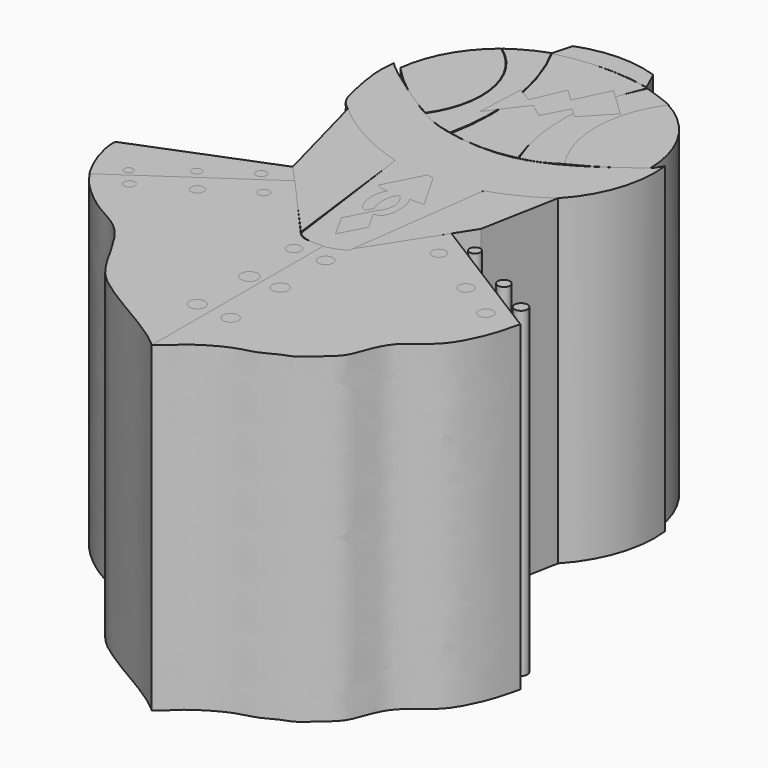
from build123d import *

# Parameters (mm, degrees)
F13_DEPTH = 50.8
F3_R      = 0.8258639316
F3_R_2    = 0.764978056
F3_R_3    = 0.6797787927
F3_R_4    = 0.8640740481
F3_R_5    = 0.9923388608
F3_R_6    = 0.8490565484
F3_R_7    = 1.1012910221
F3_R_8    = 1.1556611148
F3_R_9    = 1.2502681644
F3_R_10   = 1.3249013173
F3_R_11   = 1.1898830125
F3_R_12   = 1.2566568943
F3_R_13   = 0.8479964072
F3_R_14   = 1.0809877486
F3_R_15   = 1.1534001033
F3_R_16   = 0.9668649048
F3_R_17   = 1.0273458698
F3_R_18   = 1.137706782


# Not quite as in the source:
# - a feature of the source that left no trace in its solid (it failed there, or was rolled back) is left out


with BuildPart() as f13:
    # F9 (on Top) → F13 (new body)
    with BuildSketch(Plane.XY):
        with BuildLine():
            add(Edge.make_bspline(
                [(-21.125846708, 27.3723586698), (-20.8347521232, 27.1254879671), (-20.5297161329, 26.8714296714), (-20.2117994559, 26.6140409524)],
                knots=[0, 0, 0, 0, 0.031945991, 0.031945991, 0.031945991, 0.031945991], degree=3))
            ThreePointArc((-21.125846708, 27.3723586698), (-21.3344056847, 24.3224414992), (-20.8773446183, 21.2997627574))
            add(Edge.make_bspline(
                [(-20.8773446183, 21.2997627574), (-20.6619361674, 20.9767399348), (-20.4394229312, 20.6837653222), (-20.2117994559, 20.4157030891)],
                knots=[0, 0, 0, 0, 0.0250038431, 0.0250038431, 0.0250038431, 0.0250038431], degree=3))
            Line((-20.2117994559, 20.4157030891), (-20.2117994559, 26.6140409524))
        make_face()
        with BuildLine():
            add(Edge.make_bspline(
                [(-20.2117994559, 26.6140409524), (-19.904375261, 26.3651470584), (-19.5849065742, 26.1131389472), (-19.2543525186, 25.8615043496)],
                knots=[0.031945991, 0.031945991, 0.031945991, 0.031945991, 0.0628376406, 0.0628376406, 0.0628376406, 0.0628376406], degree=3))
            Line((-20.2117994559, 26.6140409524), (-20.2117994559, 20.4157030891))
            add(Edge.make_bspline(
                [(-20.2117994559, 20.4157030891), (-19.900507453, 20.0491080825), (-19.5796579779, 19.7291056859), (-19.2543525186, 19.4425598906)],
                knots=[0.0250038431, 0.0250038431, 0.0250038431, 0.0250038431, 0.059198455, 0.059198455, 0.059198455, 0.059198455], degree=3))
            Line((-19.2543525186, 19.4425598906), (-19.2543525186, 25.8615043496))
        make_face()
        with BuildLine():
            add(Edge.make_bspline(
                [(-19.2543525186, 25.8615043496), (-18.8314593105, 25.5395764818), (-18.3904223718, 25.2182599541), (-17.9332500512, 24.9048578725)],
                knots=[0.0628376406, 0.0628376406, 0.0628376406, 0.0628376406, 0.1023587675, 0.1023587675, 0.1023587675, 0.1023587675], degree=3))
            Line((-19.2543525186, 25.8615043496), (-19.2543525186, 19.4425598906))
            add(Edge.make_bspline(
                [(-19.2543525186, 19.4425598906), (-18.817899269, 19.0581093996), (-18.3734248739, 18.7338835997), (-17.9332500512, 18.4381574226)],
                knots=[0.059198455, 0.059198455, 0.059198455, 0.059198455, 0.1050764107, 0.1050764107, 0.1050764107, 0.1050764107], degree=3))
            Line((-17.9332500512, 18.4381574226), (-17.9332500512, 24.9048578725))
        make_face()
        with BuildLine():
            add(Edge.make_bspline(
                [(-17.9332500512, 24.9048578725), (-17.3830906612, 24.5277110282), (-16.8095646212, 24.1620255855), (-16.2161719054, 23.8205287606)],
                knots=[0.1023587675, 0.1023587675, 0.1023587675, 0.1023587675, 0.1499183376, 0.1499183376, 0.1499183376, 0.1499183376], degree=3))
            Line((-17.9332500512, 24.9048578725), (-17.9332500512, 18.4381574226))
            add(Edge.make_bspline(
                [(-17.9332500512, 18.4381574226), (-17.6086585708, 18.2200845282), (-17.0105720145, 17.8441146508), (-16.4375567591, 17.4777070139), (-16.1744944867, 17.3109124212)],
                knots=[0.1050764107, 0.1050764107, 0.1050764107, 0.1050764107, 0.1389074997, 0.1678652471, 0.1678652471, 0.1678652471, 0.1678652471], degree=3))
            Line((-16.1744944867, 17.3109124212), (-16.2161719054, 23.8205287606))
        make_face()
        with BuildLine():
            add(Edge.make_bspline(
                [(-16.2161719054, 23.8205287606), (-16.0014371982, 23.6969491837), (-15.5601814874, 23.452478006), (-15.1088853591, 23.2235501025), (-14.8776807746, 23.1111352228)],
                knots=[0.1499183376, 0.1499183376, 0.1499183376, 0.1499183376, 0.1671290147, 0.1848609969, 0.1848609969, 0.1848609969, 0.1848609969], degree=3))
            Line((-16.2161719054, 23.8205287606), (-16.1744944867, 17.3109124212))
            add(Edge.make_bspline(
                [(-16.1744944867, 17.3109124212), (-15.7449865853, 17.0385830032), (-15.3186992984, 16.7720913944), (-14.8776807746, 16.5121166992)],
                knots=[0.1678652471, 0.1678652471, 0.1678652471, 0.1678652471, 0.215145236, 0.215145236, 0.215145236, 0.215145236], degree=3))
            Line((-14.8776807746, 16.5121166992), (-14.8776807746, 23.1111352228))
        make_face()
        with BuildLine():
            add(Edge.make_bspline(
                [(-14.8776807746, 23.1111352228), (-14.3070567596, 22.8336899024), (-13.7230922448, 22.5791279001), (-13.1317322997, 22.3437527448)],
                knots=[0.1848609969, 0.1848609969, 0.1848609969, 0.1848609969, 0.2286243804, 0.2286243804, 0.2286243804, 0.2286243804], degree=3))
            Line((-14.8776807746, 23.1111352228), (-14.8776807746, 16.5121166992))
            add(Edge.make_bspline(
                [(-14.8776807746, 16.5121166992), (-14.4636429412, 16.2680467708), (-13.8984861896, 15.9526259429), (-13.2845672983, 15.648250525), (-13.1317322997, 15.574692191)],
                knots=[0.215145236, 0.215145236, 0.215145236, 0.215145236, 0.2595327234, 0.2738913967, 0.2738913967, 0.2738913967, 0.2738913967], degree=3))
            Line((-13.1317322997, 15.574692191), (-13.1317322997, 22.3437527448))
        make_face()
        with BuildLine():
            add(Edge.make_bspline(
                [(-13.1317322997, 22.3437527448), (-12.5834968737, 22.1255421615), (-12.0289053022, 21.9238220846), (-11.4726945758, 21.7356471914)],
                knots=[0.2286243804, 0.2286243804, 0.2286243804, 0.2286243804, 0.2691963491, 0.2691963491, 0.2691963491, 0.2691963491], degree=3))
            Line((-13.1317322997, 22.3437527448), (-13.1317322997, 15.574692191))
            add(Edge.make_bspline(
                [(-13.1317322997, 15.574692191), (-12.6094536829, 15.3233234257), (-12.0546922141, 15.0817263388), (-11.4726945758, 14.8569610447)],
                knots=[0.2738913967, 0.2738913967, 0.2738913967, 0.2738913967, 0.3229588757, 0.3229588757, 0.3229588757, 0.3229588757], degree=3))
            Line((-11.4726945758, 14.8569610447), (-11.4726945758, 21.7356471914))
        make_face()
        with BuildLine():
            add(Edge.make_bspline(
                [(-11.4726945758, 21.7356471914), (-10.8241176286, 21.5162233436), (-10.1733391103, 21.3152169328), (-9.5278695226, 21.1279581478)],
                knots=[0.2691963491, 0.2691963491, 0.2691963491, 0.2691963491, 0.3165058352, 0.3165058352, 0.3165058352, 0.3165058352], degree=3))
            Line((-11.4726945758, 21.7356471914), (-11.4726945758, 14.8569610447))
            add(Edge.make_bspline(
                [(-11.4726945758, 14.8569610447), (-10.853171685, 14.6177036395), (-10.2027872041, 14.3975185158), (-9.5278695226, 14.2049213694)],
                knots=[0.3229588757, 0.3229588757, 0.3229588757, 0.3229588757, 0.3751900608, 0.3751900608, 0.3751900608, 0.3751900608], degree=3))
            Line((-9.5278695226, 14.2049213694), (-9.5278695226, 21.1279581478))
        make_face()
        with BuildLine():
            add(Edge.make_bspline(
                [(-9.5278695226, 21.1279581478), (-9.1488679975, 21.0180050742), (-8.5926706461, 20.862851759), (-8.0437599408, 20.7159498258), (-7.8676519915, 20.6696810568)],
                knots=[0.3165058352, 0.3165058352, 0.3165058352, 0.3165058352, 0.3442846302, 0.3574699751, 0.3574699751, 0.3574699751, 0.3574699751], degree=3))
            Line((-9.5278695226, 21.1279581478), (-9.5278695226, 14.2049213694))
            add(Edge.make_bspline(
                [(-9.5278695226, 14.2049213694), (-9.2039090788, 14.1124747514), (-8.6556599801, 13.9692796344), (-8.0937090418, 13.8462753142), (-7.8676519915, 13.8003926225)],
                knots=[0.3751900608, 0.3751900608, 0.3751900608, 0.3751900608, 0.4002610263, 0.4168909002, 0.4168909002, 0.4168909002, 0.4168909002], degree=3))
            Line((-7.8676519915, 13.8003926225), (-7.8676519915, 20.6696810568))
        make_face()
        with BuildLine():
            add(Edge.make_bspline(
                [(-7.8676519915, 20.6696810568), (-7.4364796265, 20.5563993186), (-7.0087411364, 20.449203879), (-6.5817643521, 20.3504497102)],
                knots=[0.3574699751, 0.3574699751, 0.3574699751, 0.3574699751, 0.3897521995, 0.3897521995, 0.3897521995, 0.3897521995], degree=3))
            Line((-7.8676519915, 20.6696810568), (-7.8676519915, 13.8003926225))
            add(Edge.make_bspline(
                [(-7.8676519915, 13.8003926225), (-7.2935890267, 13.6838753365), (-6.7069076556, 13.5878021605), (-6.1112494197, 13.511504583)],
                knots=[0.4168909002, 0.4168909002, 0.4168909002, 0.4168909002, 0.459121809, 0.459121809, 0.459121809, 0.459121809], degree=3))
            Line((-6.1112494197, 13.511504583), (-6.5817643521, 20.3504497102))
        make_face()
        with BuildLine():
            add(Edge.make_bspline(
                [(-6.5817643521, 20.3504497102), (-6.0578024629, 20.22926415), (-5.5349876125, 20.1207901455), (-5.0083818106, 20.0293795287)],
                knots=[0.3897521995, 0.3897521995, 0.3897521995, 0.3897521995, 0.4293671292, 0.4293671292, 0.4293671292, 0.4293671292], degree=3))
            Line((-6.5817643521, 20.3504497102), (-6.1112494197, 13.511504583))
            add(Edge.make_bspline(
                [(-6.1112494197, 13.511504583), (-5.62787322, 13.4495891576), (-5.1385854764, 13.4006965769), (-4.6453322191, 13.3644695901)],
                knots=[0.459121809, 0.459121809, 0.459121809, 0.459121809, 0.493392159, 0.493392159, 0.493392159, 0.493392159], degree=3))
            Line((-4.6453322191, 13.3644695901), (-5.0083818106, 20.0293795287))
        make_face()
        with BuildLine():
            add(Edge.make_bspline(
                [(-5.0083818106, 20.0293795287), (-4.4190508025, 19.927080787), (-3.8249719601, 19.846152441), (-3.2192242461, 19.7926939744)],
                knots=[0.4293671292, 0.4293671292, 0.4293671292, 0.4293671292, 0.4737006826, 0.4737006826, 0.4737006826, 0.4737006826], degree=3))
            Line((-5.0083818106, 20.0293795287), (-4.6453322191, 13.3644695901))
            add(Edge.make_bspline(
                [(-4.6453322191, 13.3644695901), (-4.0948822571, 13.3240417912), (-3.5394937933, 13.2993872473), (-2.9818713665, 13.2900094613)],
                knots=[0.493392159, 0.493392159, 0.493392159, 0.493392159, 0.5316364333, 0.5316364333, 0.5316364333, 0.5316364333], degree=3))
            Line((-2.9818713665, 13.2900094613), (-3.2192242461, 19.7926939744))
        make_face()
        with BuildLine():
            add(Edge.make_bspline(
                [(-3.2192242461, 19.7926939744), (-2.6894172346, 19.7459374292), (-2.1506837335, 19.7201948771), (-1.5983930182, 19.719547358)],
                knots=[0.4737006826, 0.4737006826, 0.4737006826, 0.4737006826, 0.5124762766, 0.5124762766, 0.5124762766, 0.5124762766], degree=3))
            Line((-3.2192242461, 19.7926939744), (-2.9818713665, 13.2900094613))
            add(Edge.make_bspline(
                [(-2.9818713665, 13.2900094613), (-2.598295297, 13.2835586909), (-2.0336888013, 13.2847004629), (-1.4687014205, 13.3010698813), (-1.288695996, 13.3077850564)],
                knots=[0.5316364333, 0.5316364333, 0.5316364333, 0.5316364333, 0.5579438193, 0.5702532866, 0.5702532866, 0.5702532866, 0.5702532866], degree=3))
            Line((-1.288695996, 13.3077850564), (-1.5983930182, 19.719547358))
        make_face()
        with BuildLine():
            add(Edge.make_bspline(
                [(-1.5983930182, 19.719547358), (-1.0760239175, 19.7189349198), (-0.541526796, 19.7407720111), (0, 19.7822179046)],
                knots=[0.5124762766, 0.5124762766, 0.5124762766, 0.5124762766, 0.549151114, 0.549151114, 0.549151114, 0.549151114], degree=3))
            Line((-1.5983930182, 19.719547358), (-1.288695996, 13.3077850564))
            add(Edge.make_bspline(
                [(-1.288695996, 13.3077850564), (-0.7545655199, 13.3277110099), (-0.2212218042, 13.3608203078), (0.3079894723, 13.4058075855)],
                knots=[0.5702532866, 0.5702532866, 0.5702532866, 0.5702532866, 0.6067791948, 0.6067791948, 0.6067791948, 0.6067791948], degree=3))
            Line((0.3079894723, 13.4058075855), (0, 19.7822179046))
        make_face()
        with BuildLine():
            add(Edge.make_bspline(
                [(0, 19.7822179046), (0.5137068711, 19.8215345929), (1.0337396967, 19.878497104), (1.5557462092, 19.950680415)],
                knots=[0.549151114, 0.549151114, 0.549151114, 0.549151114, 0.5839418503, 0.5839418503, 0.5839418503, 0.5839418503], degree=3))
            Line((0, 19.7822179046), (0.3079894723, 13.4058075855))
            add(Edge.make_bspline(
                [(0.3079894723, 13.4058075855), (0.7270533852, 13.4414314383), (1.143526051, 13.4845033813), (1.5557462092, 13.5343752499)],
                knots=[0.6067791948, 0.6067791948, 0.6067791948, 0.6067791948, 0.6357027849, 0.6357027849, 0.6357027849, 0.6357027849], degree=3))
            Line((1.5557462092, 13.5343752499), (1.5557462092, 19.950680415))
        make_face()
        with BuildLine():
            add(Edge.make_bspline(
                [(1.5557462092, 19.950680415), (2.0910865169, 20.0247075295), (2.6285026284, 20.1147429555), (3.16330017, 20.2181710532)],
                knots=[0.5839418503, 0.5839418503, 0.5839418503, 0.5839418503, 0.6196212585, 0.6196212585, 0.6196212585, 0.6196212585], degree=3))
            Line((1.5557462092, 19.950680415), (1.5557462092, 13.5343752499))
            add(Edge.make_bspline(
                [(1.5557462092, 13.5343752499), (2.1002950478, 13.6002567153), (2.6374229225, 13.6780045916), (3.16330017, 13.7661246805)],
                knots=[0.6357027849, 0.6357027849, 0.6357027849, 0.6357027849, 0.673911269, 0.673911269, 0.673911269, 0.673911269], degree=3))
            Line((3.16330017, 13.7661246805), (3.16330017, 20.2181710532))
        make_face()
        with BuildLine():
            add(Edge.make_bspline(
                [(3.16330017, 20.2181710532), (3.8146725961, 20.3441443529), (4.4621604418, 20.4899853328), (5.0972817207, 20.6509679486)],
                knots=[0.6196212585, 0.6196212585, 0.6196212585, 0.6196212585, 0.6630780453, 0.6630780453, 0.6630780453, 0.6630780453], degree=3))
            Line((3.16330017, 20.2181710532), (3.16330017, 13.7661246805))
            add(Edge.make_bspline(
                [(3.16330017, 13.7661246805), (3.7296270842, 13.8610228308), (4.2829060457, 13.9679501896), (4.818353959, 14.0850405636)],
                knots=[0.673911269, 0.673911269, 0.673911269, 0.673911269, 0.7150586908, 0.7150586908, 0.7150586908, 0.7150586908], degree=3))
            Line((4.818353959, 14.0850405636), (5.0972817207, 20.6509679486))
        make_face()
        with BuildLine():
            add(Edge.make_bspline(
                [(5.0972817207, 20.6509679486), (5.58535494, 20.7746786573), (6.0661250841, 20.9073312582), (6.5357428463, 21.0467809712)],
                knots=[0.6630780453, 0.6630780453, 0.6630780453, 0.6630780453, 0.6964733896, 0.6964733896, 0.6964733896, 0.6964733896], degree=3))
            Line((5.0972817207, 20.6509679486), (4.818353959, 14.0850405636))
            add(Edge.make_bspline(
                [(4.818353959, 14.0850405636), (5.3750991504, 14.2067881717), (5.9125666354, 14.3395233348), (6.4412617638, 14.4826543305)],
                knots=[0.7150586908, 0.7150586908, 0.7150586908, 0.7150586908, 0.7578427388, 0.7578427388, 0.7578427388, 0.7578427388], degree=3))
            Line((6.4412617638, 14.4826543305), (6.5357428463, 21.0467809712))
        make_face()
        with BuildLine():
            add(Edge.make_bspline(
                [(6.5357428463, 21.0467809712), (7.1170989648, 21.2194106083), (7.6813642554, 21.4024566995), (8.2282215408, 21.5939352841)],
                knots=[0.6964733896, 0.6964733896, 0.6964733896, 0.6964733896, 0.7378146449, 0.7378146449, 0.7378146449, 0.7378146449], degree=3))
            Line((6.5357428463, 21.0467809712), (6.4412617638, 14.4826543305))
            add(Edge.make_bspline(
                [(6.4412617638, 14.4826543305), (6.9056378419, 14.6083725504), (7.3632461539, 14.7421110284), (7.8212054558, 14.8834687947)],
                knots=[0.7578427388, 0.7578427388, 0.7578427388, 0.7578427388, 0.7954218413, 0.7954218413, 0.7954218413, 0.7954218413], degree=3))
            Line((7.8212054558, 14.8834687947), (8.2282215408, 21.5939352841))
        make_face()
        with BuildLine():
            add(Edge.make_bspline(
                [(8.2282215408, 21.5939352841), (8.6633628548, 21.746297235), (9.0874821375, 21.9039982932), (9.500419591, 22.0660389143)],
                knots=[0.7378146449, 0.7378146449, 0.7378146449, 0.7378146449, 0.7707104087, 0.7707104087, 0.7707104087, 0.7707104087], degree=3))
            Line((8.2282215408, 21.5939352841), (7.8212054558, 14.8834687947))
            add(Edge.make_bspline(
                [(7.8212054558, 14.8834687947), (8.5874074933, 15.1199714884), (9.6396761943, 15.4736113373), (10.7565133697, 15.8638421146), (11.0588213429, 15.9738352262)],
                knots=[0.7954218413, 0.7954218413, 0.7954218413, 0.7954218413, 0.8582946442, 0.881658047, 0.881658047, 0.881658047, 0.881658047], degree=3))
            Line((11.0588213429, 15.9738352262), (11.0588213429, 22.7200354778))
            add(Edge.make_bspline(
                [(9.500419591, 22.0660389143), (10.0390285895, 22.2773942561), (10.5586140402, 22.4961324584), (11.0588213429, 22.7200354778)],
                knots=[0.7707104087, 0.7707104087, 0.7707104087, 0.7707104087, 0.8136175228, 0.8136175228, 0.8136175228, 0.8136175228], degree=3))
        make_face()
        with BuildLine():
            Line((11.0588213429, 22.7200354778), (11.0588213429, 15.9738352262))
            add(Edge.make_bspline(
                [(11.0588213429, 15.9738352262), (11.5241048545, 16.1431261011), (11.9887504135, 16.3225330625), (12.434497183, 16.5178338427)],
                knots=[0.881658047, 0.881658047, 0.881658047, 0.881658047, 0.9176167616, 0.9176167616, 0.9176167616, 0.9176167616], degree=3))
            Line((12.434497183, 16.5178338427), (12.6337970085, 23.4722221968))
            add(Edge.make_bspline(
                [(11.0588213429, 22.7200354778), (11.6072647333, 22.9655299566), (12.1324124203, 23.2172333904), (12.6337970085, 23.4722221968)],
                knots=[0.8136175228, 0.8136175228, 0.8136175228, 0.8136175228, 0.8606622641, 0.8606622641, 0.8606622641, 0.8606622641], degree=3))
        make_face()
        with BuildLine():
            Line((12.6337970085, 23.4722221968), (12.434497183, 16.5178338427))
            add(Edge.make_bspline(
                [(12.434497183, 16.5178338427), (12.8998213773, 16.7217123326), (13.3445502373, 16.9429114299), (13.7479096275, 17.1880040753)],
                knots=[0.9176167616, 0.9176167616, 0.9176167616, 0.9176167616, 0.9551548011, 0.9551548011, 0.9551548011, 0.9551548011], degree=3))
            Line((13.7479096275, 17.1880040753), (14.17928578, 24.3000945385))
            add(Edge.make_bspline(
                [(12.6337970085, 23.4722221968), (13.1713354673, 23.7455977515), (13.6815602475, 24.0227495651), (14.17928578, 24.3000945385)],
                knots=[0.8606622641, 0.8606622641, 0.8606622641, 0.8606622641, 0.9110993104, 0.9110993104, 0.9110993104, 0.9110993104], degree=3))
        make_face()
        with BuildLine():
            Line((14.17928578, 24.3000945385), (13.7479096275, 17.1880040753))
            add(Edge.make_bspline(
                [(13.7479096275, 17.1880040753), (14.2297870054, 17.4808064848), (14.6526213462, 17.8077100721), (14.980992038, 18.179921926)],
                knots=[0.9551548011, 0.9551548011, 0.9551548011, 0.9551548011, 1, 1, 1, 1], degree=3))
            Line((14.980992038, 18.179921926), (15.3937334453, 24.9847816969))
            add(Edge.make_bspline(
                [(14.17928578, 24.3000945385), (14.5898345398, 24.5288624587), (14.9918790985, 24.7577618003), (15.3937334453, 24.9847816969)],
                knots=[0.9110993104, 0.9110993104, 0.9110993104, 0.9110993104, 0.9527022933, 0.9527022933, 0.9527022933, 0.9527022933], degree=3))
        make_face()
        with BuildLine():
            Line((15.3937334453, 24.9847816969), (14.980992038, 18.179921926))
            ThreePointArc((14.980992038, 18.179921926), (16.5063806562, 21.8154594304), (16.7757962894, 25.7488242238))
            add(Edge.make_bspline(
                [(15.3937334453, 24.9847816969), (15.8505946536, 25.2428766637), (16.3072100126, 25.4985424439), (16.7757962894, 25.7488242238)],
                knots=[0.9527022933, 0.9527022933, 0.9527022933, 0.9527022933, 1, 1, 1, 1], degree=3))
        make_face()
    extrude(amount=F13_DEPTH)


with BuildPart() as f13b:
    # F8 (on Top) → F13, piece 2 (new body)
    with BuildSketch(Plane.XY):
        with BuildLine():
            ThreePointArc((-12.3988108372, 23.6741252104), (-10.1171786146, 33.994784483), (-15.8344633881, 42.8849199285))
            ThreePointArc((-15.8344633881, 42.8849199285), (-20.2435563178, 37.6436153683), (-22.3273675175, 31.1191150167))
            ThreePointArc((-22.3273675175, 31.1191150167), (-17.6977421328, 26.9503306057), (-12.3988108372, 23.6741252104))
        make_face()
    extrude(amount=F13_DEPTH)


with BuildPart() as f13c:
    # F8 (on Top) → F13, piece 3 (new body)
    with BuildSketch(Plane.XY):
        with BuildLine():
            ThreePointArc((9.5350146294, 44.1038645804), (6.257298337, 33.888541162), (9.5350146294, 23.6732177436))
            ThreePointArc((9.5350146294, 23.6732177436), (14.177280096, 26.3004344114), (18.5024803593, 29.4222189595))
            ThreePointArc((18.5024803593, 29.4222189595), (16.0429971981, 37.999441988), (9.5350146294, 44.1038645804))
        make_face()
    extrude(amount=F13_DEPTH)


with BuildPart() as f13d:
    # F8 (on Top) → F13, piece 4 (new body)
    with BuildSketch(Plane.XY):
        with BuildLine():
            ThreePointArc((-10.1647363602, 45.9095185055), (-6.1837471128, 33.9589399996), (-6.5014758147, 21.3667340577))
            ThreePointArc((-6.5014758147, 21.3667340577), (-1.2340764428, 20.7648960213), (4.0342169814, 21.3588569313))
            ThreePointArc((4.0342169814, 21.3588569313), (2.0273038958, 33.7407666562), (4.8860239137, 45.9541653817))
            ThreePointArc((4.8860239137, 45.9541653817), (-2.6417550196, 46.7404922067), (-10.1647363602, 45.9095185055))
        make_face()
    extrude(amount=F13_DEPTH)


with BuildPart() as f13e:
    # F7 (on Top) → F13, piece 5 (new body)
    with BuildSketch(Plane.XY):
        with BuildLine():
            ThreePointArc((-12.3944459483, 23.4615169466), (-9.6503858131, 22.2226681718), (-6.7442338914, 21.4359704405))
            ThreePointArc((-6.7442338914, 21.4359704405), (-6.2858776286, 33.9589836539), (-10.2293472737, 45.8537302911))
            ThreePointArc((-10.2293472737, 45.8537302911), (-13.0947819539, 44.6092461951), (-15.7425962389, 42.951375246))
            ThreePointArc((-15.7425962389, 42.951375246), (-10.0041611915, 33.9046598841), (-12.3944459483, 23.4615169466))
        make_face()
    extrude(amount=F13_DEPTH)


with BuildPart() as f13f:
    # F7 (on Top) → F13, piece 6 (new body)
    with BuildSketch(Plane.XY):
        with BuildLine():
            ThreePointArc((9.7108701983, 44.0882421106), (7.3439136897, 45.0182369237), (4.9339610864, 45.8303341562))
            ThreePointArc((4.9339610864, 45.8303341562), (1.9006592019, 33.6722260465), (4.1810232215, 21.3506817818))
            ThreePointArc((4.1810232215, 21.3506817818), (6.9727148218, 22.2661082897), (9.5312194899, 23.7102694809))
            ThreePointArc((9.5312194899, 23.7102694809), (6.4216220228, 33.9274616721), (9.7108701983, 44.0882421106))
        make_face()
    extrude(amount=F13_DEPTH)


with BuildPart() as f13g:
    # F11 (on Top) → F13, piece 7 (new body)
    with BuildSketch(Plane.XY):
        with BuildLine():
            ThreePointArc((-7.3326835409, 11.3885579631), (-14.377405186, 14.2696952056), (-20.5801893026, 18.6804234982))
            Line((-20.5801893026, 18.6804234982), (-16.1750596017, 2.1767148282))
            Line((-16.1750596017, 2.1767148282), (-4.507355392, -10.7746338472))
            Line((-4.507355392, -10.7746338472), (-7.3326835409, 11.3885579631))
        make_face()
    extrude(amount=F13_DEPTH)


with BuildPart() as f13h:
    # F11 (on Top) → F13, piece 8 (new body)
    with BuildSketch(Plane.XY):
        with BuildLine():
            Line((6.2384190969, 11.8528539315), (3.1280014664, -10.5955125764))
            Line((3.1280014664, -10.5955125764), (12.3193198815, 3.711481113))
            Line((12.3193198815, 3.711481113), (14.6430647001, 16.0904526711))
            ThreePointArc((14.6430647001, 16.0904526711), (10.586652774, 13.6822608237), (6.2384190969, 11.8528539315))
        make_face()
    extrude(amount=F13_DEPTH)


with BuildPart() as f13i:
    # F6 (on Top) → F13, piece 9 (new body)
    with BuildSketch(Plane.XY):
        with BuildLine():
            add(Edge.make_bspline(
                [(0, -12.0247779414), (0.5012354918, -11.9426944258), (1.7908691638, -11.7338985108), (2.6501969117, -11.1655605144), (3.1240915414, -10.5731924996)],
                knots=[0, 0, 0, 0, 0.492792412, 1, 1, 1, 1], degree=3))
            Line((0, -12.0247779414), (0, -45.9450371563))
            add(Edge.make_bspline(
                [(32.0461690426, -13.1501732394), (31.7097565093, -14.5282364317), (31.0642043992, -17.3739063034), (28.646181352, -22.4797561646), (26.1181511575, -24.640107946), (22.9830511449, -26.8576842658), (21.4926242295, -30.1016614383), (20.5465442347, -33.3459081143), (17.8988820449, -35.3011340828), (15.9446171515, -37.3481670644), (13.8112930921, -37.899895011), (11.542638481, -39.3912219109), (8.5051505152, -39.9352404708), (5.444791947, -41.5575600393), (2.4923123567, -43.5404964495), (1.700661544, -44.6719397288), (0, -45.9450371563)],
                knots=[0, 0, 0, 0, 0.0814586936, 0.1723459536, 0.2433655723, 0.3178750274, 0.3907644345, 0.4610811587, 0.5307268637, 0.5952181363, 0.6517409884, 0.7147459782, 0.782686328, 0.8556077005, 0.924329985, 1, 1, 1, 1], degree=3))
            Line((32.0461690426, -13.1501732394), (10.2511029691, 0.4863103968))
            Line((10.2511029691, 0.4863103968), (3.1240915414, -10.5731924996))
        make_face()
    extrude(amount=F13_DEPTH)


with BuildPart() as f13j:
    # F12 (on Top) → F13, piece 10 (new body)
    with BuildSketch(Plane.XY):
        with BuildLine():
            add(Edge.make_bspline(
                [(-23.7491764128, 31.6212512553), (-23.5014987322, 31.3483771554), (-22.5627618935, 30.3140691193), (-12.0611662049, 22.8982617788), (-7.0474683792, 21.2085651947), (5.2835711864, 19.5360643586), (14.377356866, 26.3330175771), (18.7600348145, 29.6710412949)],
                knots=[0, 0, 0, 0, 0.0861918774, 0.3258221147, 0.4937836066, 0.720934999, 1, 1, 1, 1], degree=3))
            add(Edge.make_bspline(
                [(-23.7491764128, 31.6212512553), (-23.8477742303, 30.5311013084), (-24.067282785, 28.1040979001), (-23.0487521074, 22.9537554354), (-22.3178278064, 19.9419018956), (-21.1057583084, 18.9667539886), (-20.5545537174, 18.523292616)],
                knots=[0, 0, 0, 0, 0.2545070369, 0.566609619, 0.8029100079, 1, 1, 1, 1], degree=3))
            ThreePointArc((-20.5545537174, 18.523292616), (-14.3465072066, 14.2264422516), (-7.3501081206, 11.3886324689))
            Line((-7.3501081206, 11.3886324689), (-4.3249502778, -10.8443647623))
            add(Edge.make_bspline(
                [(-4.3249502778, -10.8443647623), (-3.9669240627, -11.6108496135), (-1.9831716654, -12.1008701365), (-0.1800869966, -12.2315672406), (2.1804859454, -11.5264114101), (1.6686771996, -11.6793001071), (3.211584175, -10.8443647623)],
                knots=[0, 0, 0, 0, 0.2802837955, 0.5352435302, 0.7663564293, 1, 1, 1, 1], degree=3))
            Line((3.211584175, -10.8443647623), (6.2316702679, 11.8567077443))
            ThreePointArc((6.2316702679, 11.8567077443), (10.5869107262, 13.6279285619), (14.6170314401, 16.0493887961))
            ThreePointArc((14.6170314401, 16.0493887961), (18.7520084952, 22.9933533972), (19.5831675082, 31.0323741287))
            Line((19.5831675082, 31.0323741287), (18.7600348145, 29.6710412949))
        make_face()
    extrude(amount=F13_DEPTH)


with BuildPart() as f13k:
    # F1 (on Top) → F13, piece 11 (new body)
    with BuildSketch(Plane.XY):
        Polygon((6.5561048687, 38.4634584188), (2.0181094296, 42.7997633815), (-0.5179300206, 37.5159755349), (-2.4259227794, 39.3815711141), (-4.6731135808, 34.33545), (-7.0475041866, 35.8129740924), (-7.3556074226, 28.1221466535), (-3.2739192247, 33.5303917527), (-1.0267283069, 31.8344011903), (1.0653183376, 35.8129740924), (2.6115651192, 34.33545), align=None)
    extrude(amount=F13_DEPTH)


with BuildPart() as f13l:
    # F2 (on Top) → F13, piece 12 (new body)
    with BuildSketch(Plane.XY):
        with BuildLine():
            Line((4.6263667755, 46.0232459009), (3.2002124935, 49.1607859731))
            ThreePointArc((3.2002124935, 49.1607859731), (-3.0867123745, 50.140822554), (-9.3360953033, 48.9445328712))
            Line((-9.3360953033, 48.9445328712), (-10.2056413889, 45.7380153239))
            ThreePointArc((-10.2056413889, 45.7380153239), (-2.8065800825, 46.7616560321), (4.6263667755, 46.0232459009))
        make_face()
    extrude(amount=F13_DEPTH)


with BuildPart() as f13m:
    # F4 (on Top) → F13, piece 13 (new body)
    with BuildSketch(Plane.XY):
        with BuildLine():
            Line((-34.5214679837, -15.0747038424), (-13.6476866901, -0.6190927234))
            Line((-13.6476866901, -0.6190927234), (-16.1745920777, 2.1744580008))
            Line((-16.1745920777, 2.1744580008), (-37.4110601842, -6.274796091))
            add(Edge.make_bspline(
                [(-34.5214679837, -15.0747038424), (-34.8318337722, -14.6441931803), (-35.4131860958, -13.573033533), (-36.7515156736, -10.8689685545), (-37.5907054956, -7.3068456647), (-37.4076562249, -6.5654079293), (-37.4110601842, -6.274796091)],
                knots=[0, 0, 0, 0, 0.2169891206, 0.5159779156, 0.8345383602, 1, 1, 1, 1], degree=3))
        make_face()
    extrude(amount=F13_DEPTH)


with BuildPart() as f13n:
    # F5 (on Top) → F13, piece 14 (new body)
    with BuildSketch(Plane.XY):
        with BuildLine():
            Line((0, -45.8658896387), (0, -11.98398415))
            add(Edge.make_bspline(
                [(0, -11.98398415), (-0.757853317, -12.0691313531), (-2.2823968877, -11.9373347854), (-3.522585379, -11.98398415), (-4.4776955619, -10.8777750283)],
                knots=[0, 0, 0, 0, 0.4771596755, 1, 1, 1, 1], degree=3))
            Line((-4.4776955619, -10.8777750283), (-13.6284315959, -0.5788833369))
            Line((-13.6284315959, -0.5788833369), (-34.5914363861, -14.926860109))
            add(Edge.make_bspline(
                [(0, -45.8658896387), (-1.0862513072, -44.8902953717), (-3.5963360104, -43.0816351518), (-7.4779805105, -40.839725523), (-13.8657304028, -37.0070267492), (-16.9276314083, -34.3148966756), (-19.6071658184, -29.5579111833), (-22.7281685987, -23.9817210793), (-27.1986720795, -21.8033968956), (-29.9162115543, -19.9481899875), (-32.9156425637, -17.3024699024), (-34.0417535859, -15.6896636097), (-34.5914363861, -14.926860109)],
                knots=[0, 0, 0, 0, 0.0976146874, 0.1981798717, 0.3239604974, 0.4180537563, 0.5254412879, 0.6429781982, 0.744207795, 0.8290483984, 0.9208484418, 1, 1, 1, 1], degree=3))
        make_face()
    extrude(amount=F13_DEPTH)


with BuildPart() as f13o:
    # F3 (on Top) → F13, piece 15 (new body)
    with BuildSketch(Plane.XY):
        with Locations((-18.0757213384, -1.6571147135)):
            Circle(F3_R)
    extrude(amount=F13_DEPTH)


with BuildPart() as f13p:
    # F3 (on Top) → F13, piece 16 (new body)
    with BuildSketch(Plane.XY):
        with Locations((-24.6791169047, -6.1492202803)):
            Circle(F3_R_2)
    extrude(amount=F13_DEPTH)


with BuildPart() as f13q:
    # F3 (on Top) → F13, piece 17 (new body)
    with BuildSketch(Plane.XY):
        with Locations((-31.4172767103, -11.1803784966)):
            Circle(F3_R_3)
    extrude(amount=F13_DEPTH)


with BuildPart() as f13r:
    # F3 (on Top) → F13, piece 18 (new body)
    with BuildSketch(Plane.XY):
        with Locations((-14.6617209539, -5.4330052808)):
            Circle(F3_R_4)
    extrude(amount=F13_DEPTH)


with BuildPart() as f13s:
    # F3 (on Top) → F13, piece 19 (new body)
    with BuildSketch(Plane.XY):
        with Locations((-21.5795636177, -9.8801897839)):
            Circle(F3_R_5)
    extrude(amount=F13_DEPTH)


with BuildPart() as f13t:
    # F3 (on Top) → F13, piece 20 (new body)
    with BuildSketch(Plane.XY):
        with Locations((-29.0500540286, -13.9810964465)):
            Circle(F3_R_6)
    extrude(amount=F13_DEPTH)


with BuildPart() as f13u:
    # F3 (on Top) → F13, piece 21 (new body)
    with BuildSketch(Plane.XY):
        with Locations((-2.3890119046, -14.7747769952)):
            Circle(F3_R_7)
    extrude(amount=F13_DEPTH)


with BuildPart() as f13v:
    # F3 (on Top) → F13, piece 22 (new body)
    with BuildSketch(Plane.XY):
        with Locations((2.6325094514, -14.8281967267)):
            Circle(F3_R_8)
    extrude(amount=F13_DEPTH)


with BuildPart() as f13w:
    # F3 (on Top) → F13, piece 23 (new body)
    with BuildSketch(Plane.XY):
        with Locations((2.7871238999, -23.9913351834)):
            Circle(F3_R_9)
    extrude(amount=F13_DEPTH)


with BuildPart() as f13x:
    # F3 (on Top) → F13, piece 24 (new body)
    with BuildSketch(Plane.XY):
        with Locations((-2.0236198325, -24.0479316562)):
            Circle(F3_R_10)
    extrude(amount=F13_DEPTH)


with BuildPart() as f13y:
    # F3 (on Top) → F13, piece 25 (new body)
    with BuildSketch(Plane.XY):
        with Locations((3.0701088253, -34.1221950948)):
            Circle(F3_R_11)
    extrude(amount=F13_DEPTH)


with BuildPart() as f13z:
    # F3 (on Top) → F13, piece 26 (new body)
    with BuildSketch(Plane.XY):
        with Locations((-2.4197986349, -33.8392108679)):
            Circle(F3_R_12)
    extrude(amount=F13_DEPTH)


with BuildPart() as f13ba:
    # F3 (on Top) → F13, piece 27 (new body)
    with BuildSketch(Plane.XY):
        with Locations((15.3534067795, -1.2318532681)):
            Circle(F3_R_13)
    extrude(amount=F13_DEPTH)


with BuildPart() as f13bb:
    # F3 (on Top) → F13, piece 28 (new body)
    with BuildSketch(Plane.XY):
        with Locations((12.3528148979, -4.5973323286)):
            Circle(F3_R_14)
    extrude(amount=F13_DEPTH)


with BuildPart() as f13bc:
    # F3 (on Top) → F13, piece 29 (new body)
    with BuildSketch(Plane.XY):
        with Locations((20.7475516945, -9.7540998831)):
            Circle(F3_R_15)
    extrude(amount=F13_DEPTH)


with BuildPart() as f13bd:
    # F3 (on Top) → F13, piece 30 (new body)
    with BuildSketch(Plane.XY):
        with Locations((23.6446894705, -5.8888122439)):
            Circle(F3_R_16)
    extrude(amount=F13_DEPTH)


with BuildPart() as f13be:
    # F3 (on Top) → F13, piece 31 (new body)
    with BuildSketch(Plane.XY):
        with Locations((29.214899987, -9.4824964181)):
            Circle(F3_R_17)
    extrude(amount=F13_DEPTH)


with BuildPart() as f13bf:
    # F3 (on Top) → F13, piece 32 (new body)
    with BuildSketch(Plane.XY):
        with Locations((26.863720268, -13.4717701003)):
            Circle(F3_R_18)
    extrude(amount=F13_DEPTH)


with BuildPart() as f13bg:
    # F10 (on Top) → F13, piece 33 (new body)
    with BuildSketch(Plane.XY):
        Polygon((1.6604810979, 4.9493764527), (-0.8181142621, 8.7527381256), (-1.1432979159, 8.101375892), (0.8933984791, 4.9493764527), align=None)
        with BuildLine():
            Line((-1.1432979159, 8.101375892), (-0.8181142621, 8.7527381256))
            Line((-0.8181142621, 8.7527381256), (1.6604810979, 4.9493764527))
            Line((1.6604810979, 4.9493764527), (0.8933984791, 4.9493764527))
            Line((0.8933984791, 4.9493764527), (0.3661298542, 4.9493764527))
            Line((0.3661298542, 4.9493764527), (-0.708638865, 4.9493764527))
            ThreePointArc((-0.708638865, 4.9493764527), (-1.0314690423, 4.7796699658), (-1.074713287, 4.4175242074))
            Line((-1.074713287, 4.4175242074), (-0.3524365311, 4.4175242074))
            Line((-0.3524365311, 4.4175242074), (0.4958813661, 4.4175242074))
            Line((0.4958813661, 4.4175242074), (2.7894256637, 4.4175242074))
            Line((2.7894256637, 4.4175242074), (-0.7792837569, 10.663128458))
            Line((-0.7792837569, 10.663128458), (-3.9581282763, 4.4845286757))
            Line((-3.9581282763, 4.4845286757), (-2.9830893036, 4.4845286757))
            Line((-2.9830893036, 4.4845286757), (-2.7793579502, 4.4845286757))
            add(Edge.make_bspline(
                [(-2.6633592788, 5.0566024147), (-2.75964709, 4.8659111684), (-2.683070139, 4.675219922), (-2.7793579502, 4.4845286757)],
                knots=[0, 0, 0, 0, 0.583715731, 0.583715731, 0.583715731, 0.583715731], degree=3))
            Line((-2.6633592788, 5.0566024147), (-1.1432979159, 8.101375892))
        make_face()
        with BuildLine():
            Line((0.8933984791, 4.9493764527), (-1.1432979159, 8.101375892))
            Line((-1.1432979159, 8.101375892), (-2.6633592788, 5.0566024147))
            add(Edge.make_bspline(
                [(-2.6633592788, 5.0566024147), (-2.75964709, 4.8659111684), (-2.683070139, 4.675219922), (-2.7793579502, 4.4845286757)],
                knots=[0, 0, 0, 0, 0.583715731, 0.583715731, 0.583715731, 0.583715731], degree=3))
            Line((-2.7793579502, 4.4845286757), (-2.9830893036, 4.4845286757))
            add(Edge.make_bspline(
                [(-1.9819684212, -1.3112324716), (-2.25443038, -1.182075171), (-2.8576141928, -0.9140281958), (-3.3825790949, 0.3456630395), (-3.5767081191, 1.1731917465), (-3.6503566666, 2.9211241911), (-3.3301930271, 3.8522633237), (-3.0883888903, 4.28895322), (-2.9830893036, 4.4845286757)],
                knots=[0, 0, 0, 0, 0.1557604137, 0.3375743074, 0.4926518416, 0.7037976964, 0.8656182762, 1, 1, 1, 1], degree=3))
            Line((-1.9819684212, -1.3112324716), (-1.697135311, -0.7872802187))
            add(Edge.make_bspline(
                [(0.3661298542, 4.9493764527), (0.2696690591, 5.1760883101), (0.086879872, 5.6392794567), (-0.6372587321, 5.7957470786), (-1.1661976672, 5.755997952), (-1.8744977568, 4.919870221), (-2.2502969067, 4.181809682), (-2.6483083197, 2.4335962381), (-2.5852051484, 1.4594265093), (-2.4945724021, -0.2444319804), (-1.9677739763, -0.6365182418), (-1.697135311, -0.7872802187)],
                knots=[0, 0, 0, 0, 0.0949763739, 0.1867695947, 0.2669111521, 0.3796501888, 0.4869161875, 0.6339071126, 0.7516018018, 0.893187436, 1, 1, 1, 1], degree=3))
            Line((0.3661298542, 4.9493764527), (0.8933984791, 4.9493764527))
        make_face()
        with BuildLine():
            Line((-0.708638865, 4.9493764527), (0.3661298542, 4.9493764527))
            add(Edge.make_bspline(
                [(0.3661298542, 4.9493764527), (0.2696690591, 5.1760883101), (0.086879872, 5.6392794567), (-0.6372587321, 5.7957470786), (-1.1661976672, 5.755997952), (-1.8744977568, 4.919870221), (-2.2502969067, 4.181809682), (-2.6483083197, 2.4335962381), (-2.5852051484, 1.4594265093), (-2.4945724021, -0.2444319804), (-1.9677739763, -0.6365182418), (-1.697135311, -0.7872802187)],
                knots=[0, 0, 0, 0, 0.0949763739, 0.1867695947, 0.2669111521, 0.3796501888, 0.4869161875, 0.6339071126, 0.7516018018, 0.893187436, 1, 1, 1, 1], degree=3))
            Line((-1.697135311, -0.7872802187), (-1.3948566047, -0.2312366851))
            add(Edge.make_bspline(
                [(-1.074713287, 4.4175242074), (-1.1954347285, 4.2347888248), (-1.6126863313, 3.9946795481), (-2.0498827762, 1.8099173182), (-1.6021546479, 0.3130844584), (-1.3948566047, -0.2312366851)],
                knots=[0, 0, 0, 0, 0.214113771, 0.6035922949, 1, 1, 1, 1], degree=3))
            ThreePointArc((-1.074713287, 4.4175242074), (-1.0314690423, 4.7796699658), (-0.708638865, 4.9493764527))
        make_face()
        Polygon((-4.8665122614, 4.95188561), (-3.9581282763, 4.4845286757), (-0.7792837569, 10.663128458), (-1.8204441221, 10.8724129675), align=None)
        with BuildLine():
            Line((-0.3524365311, 4.4175242074), (-1.074713287, 4.4175242074))
            ThreePointArc((-1.074713287, 4.4175242074), (0.1186065752, 2.0689618817), (-0.708638865, -0.4321223378))
            add(Edge.make_bspline(
                [(-0.3524365311, 4.4175242074), (-0.1824356819, 4.2529376177), (0.0143534073, 3.9815609421), (0.57251105, 2.815666899), (0.7308017389, 1.2685734748), (0.5313322772, 0.204296783), (-0.0065083619, -0.2972542795), (-0.3667054438, -0.3920033886), (-0.708638865, -0.4321223378)],
                knots=[0, 0, 0, 0, 0.1306687541, 0.3213318156, 0.5399334952, 0.7156780678, 0.8523086513, 1, 1, 1, 1], degree=3))
        make_face()
        with BuildLine():
            Line((0.4958813661, 4.4175242074), (-0.3524365311, 4.4175242074))
            add(Edge.make_bspline(
                [(-0.3524365311, 4.4175242074), (-0.1824356819, 4.2529376177), (0.0143534073, 3.9815609421), (0.57251105, 2.815666899), (0.7308017389, 1.2685734748), (0.5313322772, 0.204296783), (-0.0065083619, -0.2972542795), (-0.3667054438, -0.3920033886), (-0.708638865, -0.4321223378)],
                knots=[0, 0, 0, 0, 0.1306687541, 0.3213318156, 0.5399334952, 0.7156780678, 0.8523086513, 1, 1, 1, 1], degree=3))
            Line((-0.708638865, -0.4321223378), (-0.5463139969, -1.5088062501))
            add(Edge.make_bspline(
                [(0.4958813661, 4.4175242074), (0.6555045423, 4.1168340595), (1.1307052174, 3.2501823966), (1.1598449918, 2.3695015118), (1.3446542777, 0.5164374507), (0.8470630233, -0.9458359589), (0.0639157508, -1.4803097059), (-0.4307431441, -1.4367241524), (-0.5463139969, -1.5088062501)],
                knots=[0, 0, 0, 0, 0.1765720057, 0.3282317132, 0.5415120943, 0.7356145537, 0.8826199019, 1, 1, 1, 1], degree=3))
        make_face()
        with BuildLine():
            Line((-0.5463139969, -1.5088062501), (-0.708638865, -0.4321223378))
            ThreePointArc((-0.708638865, -0.4321223378), (-0.7757323615, -0.5072594846), (-0.8450065791, -0.5803909474))
            Line((-0.8450065791, -0.5803909474), (-2.9603248247, -4.7166139332))
            Line((-2.9603248247, -4.7166139332), (-0.8569799829, -8.5085593164))
            Line((-0.8569799829, -8.5085593164), (1.2347623706, -4.5641311444))
            Line((1.2347623706, -4.5641311444), (-0.5463139969, -1.5088062501))
        make_face()
        Polygon((-1.2155644363, -2.7413275093), (-0.8868620498, -2.1038439061), (0.5175934639, -4.4446033426), (-0.8270979743, -6.6558732651), (-1.1259182356, -6.2375250272), (-2.2016714793, -4.5641311444), align=None, mode=Mode.SUBTRACT)
        Polygon((0.5175934639, -4.4446033426), (-0.8868620498, -2.1038439061), (-1.2155644363, -2.7413275093), (-0.2593395184, -4.325075075), (-1.1259182356, -6.2375250272), (-0.8270979743, -6.6558732651), align=None)
        Polygon((-0.2593395184, -4.325075075), (-1.2155644363, -2.7413275093), (-2.2016714793, -4.5641311444), (-1.1259182356, -6.2375250272), align=None)
    extrude(amount=F13_DEPTH)


with BuildPart() as f13bh:
    # F0 (on Top) → F13, piece 34 (new body)
    with BuildSketch(Plane.XY):
        with BuildLine():
            add(Edge.make_bspline(
                [(-29.7028111193, 21.0049106975), (-29.697978745, 20.9985442698), (-29.6931281081, 20.99216706), (-29.6882594543, 20.9857794871)],
                knots=[0, 0, 0, 0, 0.0053663437, 0.0053663437, 0.0053663437, 0.0053663437], degree=3))
            add(Edge.make_bspline(
                [(-29.6882594543, 20.9857794871), (-29.6931106459, 20.9936181089), (-29.6979619526, 21.0000093144), (-29.7028111193, 21.0049106975)],
                knots=[0.8995376411, 0.8995376411, 0.8995376411, 0.8995376411, 0.9012325725, 0.9012325725, 0.9012325725, 0.9012325725], degree=3))
        make_face()
    extrude(amount=F13_DEPTH)


solid = Compound([f13.part, f13b.part, f13c.part, f13d.part, f13e.part, f13f.part, f13g.part, f13h.part, f13i.part, f13j.part, f13k.part, f13l.part, f13m.part, f13n.part, f13o.part, f13p.part, f13q.part, f13r.part, f13s.part, f13t.part, f13u.part, f13v.part, f13w.part, f13x.part, f13y.part, f13z.part, f13ba.part, f13bb.part, f13bc.part, f13bd.part, f13be.part, f13bf.part, f13bg.part, f13bh.part])
